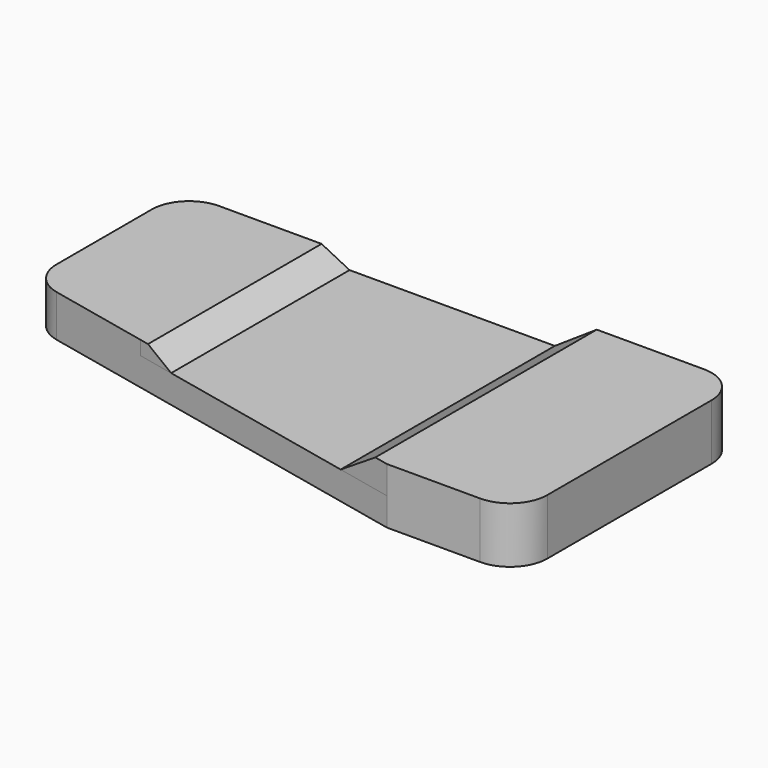
from build123d import *

# Parameters (mm, degrees)
F0_W        = 76.2
F0_H        = 38.1
F1_DEPTH    = 7.62
F4_DEPTH    = 7.621
F6_DEPTH    = 38.101
F7_T4_DEPTH = 38.1
F8_T4_DEPTH = 42.4215480701
F9_R        = 5.08


# Not quite as in the source:
# - a fillet or chamfer that OpenCascade refuses, or shapes differently, is made with other operations: its cross-section is extruded or revolved along the edge and cut away or added
# - a feature names something its author has since deleted; it is built from what else it names


with BuildPart() as f1:
    # F0 (on Top) → F1 (new body)
    with BuildSketch(Plane.XY):
        Rectangle(F0_W, F0_H)
    extrude(amount=F1_DEPTH)

    # F3 (on face) → F4 (cut, through all)
    with BuildSketch(Plane.XY.offset(7.62)):
        Polygon((-38.1, -6.35), (-38.1, -19.05), (-20.32, -19.05), (20.32, -19.05), align=None)
    extrude(amount=-F4_DEPTH, mode=Mode.SUBTRACT)

    # F5 (on face) → F6 (cut, through all)
    with BuildSketch(Plane(origin=(0, 19.05, 0), x_dir=(-1, 0, 0), z_dir=(0, 1, 0))):
        Polygon((38.1, 7.62), (-20.32, 7.62), (-20.32, 3.81), (20.32, 3.81), (20.32, 5.715), (38.1, 5.715), align=None)
    extrude(amount=-F6_DEPTH, mode=Mode.SUBTRACT)

    # F7: chamfer of 7.62 x 5.08 on 1 edges, made by hand


with BuildPart() as f7_tool2:
    # F7_s3 → F7_t4 (new body)
    with BuildSketch(Plane.XZ.offset(-19.05)):
        Polygon((20.32, 8.89), (12.7, 3.81), (20.32, 3.81), align=None)
    extrude(amount=F7_T4_DEPTH)

    split(bisect_by=Plane.XY.offset(7.62), keep=Keep.BOTTOM)

    split(bisect_by=Plane(origin=(-3.0374548736, -13.9722924188, 0), x_dir=(0, 0, 1), z_dir=(0.2124296443, 0.9771763639, 0)), keep=Keep.TOP)


with BuildPart() as f1_1:
    add(f1.part)

    # F7_t1: union F7_tool2
    add(f7_tool2.part)

    # F8: chamfer of 2.54 x 5.08 on 1 edges, made by hand


with BuildPart() as f8_tool2:
    # F8_s3 → F8_t4 (new body)
    with BuildSketch(Plane.XZ.offset(-19.05)):
        Polygon((-20.32, 6.35), (-15.24, 3.81), (-20.32, 3.81), align=None)
    extrude(amount=F8_T4_DEPTH)

    split(bisect_by=Plane.XY.offset(5.715), keep=Keep.BOTTOM)

    split(bisect_by=Plane(origin=(-3.0374548736, -13.9722924188, 0), x_dir=(0, 0, 1), z_dir=(0.2124296443, 0.9771763639, 0)), keep=Keep.TOP)


with BuildPart() as f1_2:
    add(f1_1.part)

    # F8_t1: union F8_tool2
    add(f8_tool2.part)

    # F9
    f9_edges = [f1_2.edges().sort_by_distance(p)[0] for p in [
        (-38.1, -6.35, 2.8575),
        (-38.1, 19.05, 2.8575),
        (38.1, -19.05, 3.81),
        (38.1, 19.05, 3.81),
    ]]
    fillet(f9_edges, radius=F9_R)


solid = f1_2.part
